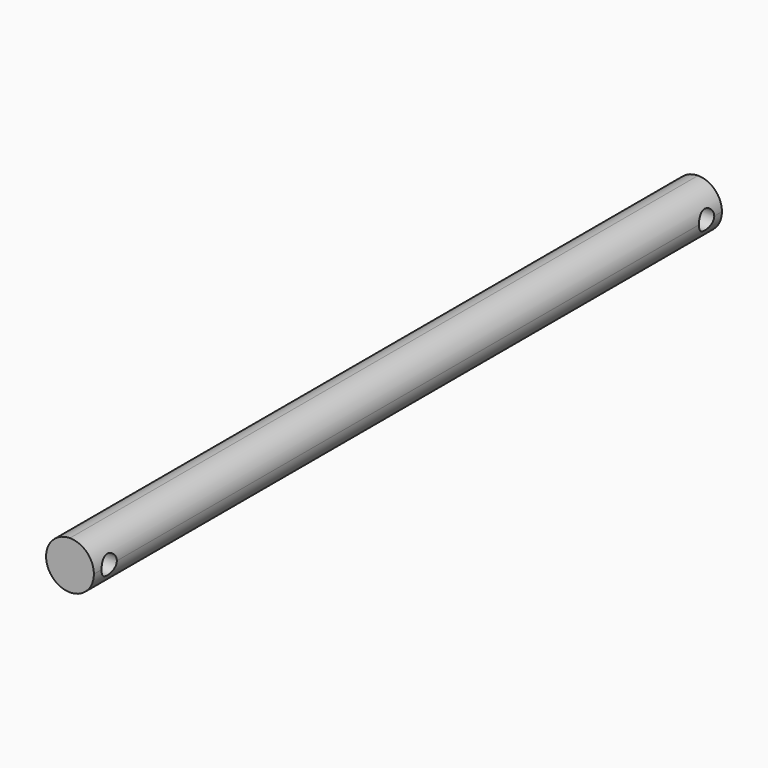
from build123d import *
from build123d import SkipClean  # not in build123d's __all__

# Parameters (mm, degrees)
F0_W     = 7.9248
F0_H     = 7.9248
F1_DEPTH = 130.175
F2_R     = 1.5875
F3_DEPTH = 25.4
F5_DEPTH = 508


with BuildPart() as f1:
    # F0 (on Front) → F1 (new body)
    with BuildSketch(Plane.XZ):
        Rectangle(F0_W, F0_H)
    extrude(amount=F1_DEPTH)

    # F2 (on face) → F3 (cut)
    with BuildSketch(Plane.YZ.offset(3.9624)):
        with BuildLine():
            ThreePointArc((-125.4125, 0), (-127, 1.5875), (-128.5875, 0))
            ThreePointArc((-128.5875, 0), (-127, -1.5875), (-125.4125, 0))
        make_face()
        with Locations((-3.175, 0)):
            Circle(F2_R)
    extrude(amount=-F3_DEPTH, mode=Mode.SUBTRACT)

    # F4 (on face) → F5 (cut)
    with BuildSketch(Plane(origin=(0, 0, 0), x_dir=(-1, 0, 0), z_dir=(0, 1, 0))):
        with BuildLine():
            ThreePointArc((-3.9624, 0), (-2.8018399098, 2.8018399098), (0, 3.9624))
            Line((0, 3.9624), (-3.9624, 3.9624))
            Line((-3.9624, 3.9624), (-3.9624, 0))
        make_face()
        with BuildLine():
            ThreePointArc((0, 3.9624), (2.8018399098, 2.8018399098), (3.9624, 0))
            Line((3.9624, 0), (3.9624, 3.9624))
            Line((3.9624, 3.9624), (0, 3.9624))
        make_face()
        with BuildLine():
            Line((3.9624, -3.9624), (3.9624, 0))
            ThreePointArc((3.9624, 0), (2.8018399098, -2.8018399098), (0, -3.9624))
            Line((0, -3.9624), (3.9624, -3.9624))
        make_face()
        with BuildLine():
            Line((-3.9624, -3.9624), (0, -3.9624))
            ThreePointArc((0, -3.9624), (-2.8018399098, -2.8018399098), (-3.9624, 0))
            Line((-3.9624, 0), (-3.9624, -3.9624))
        make_face()
    with SkipClean():  # cleaning this boolean's faces spoils the solid; the shape is the same uncleaned
        extrude(amount=-F5_DEPTH, mode=Mode.SUBTRACT)


solid = f1.part
